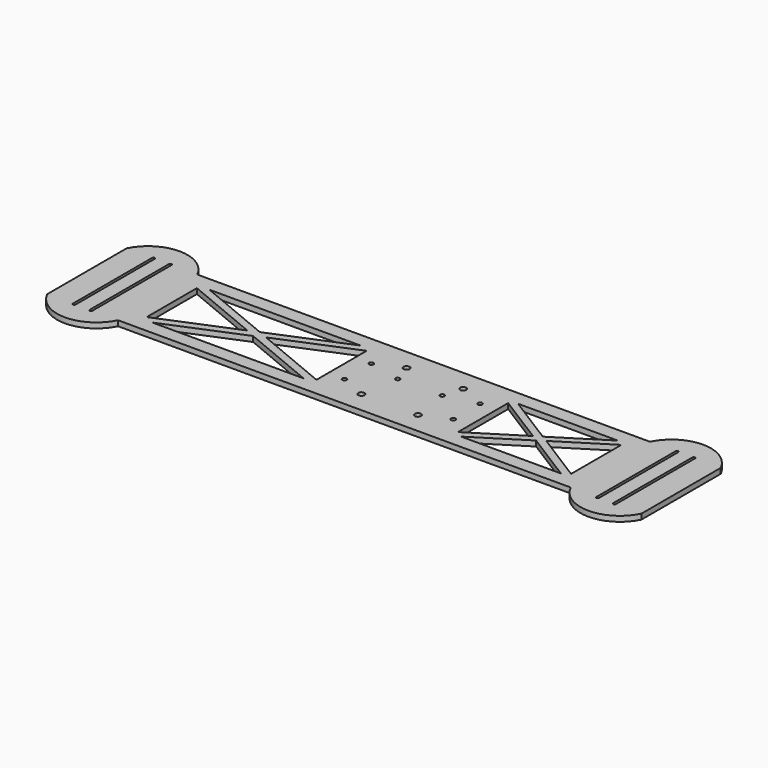
from build123d import *

# Parameters (mm, degrees)
F1_DEPTH = 4.7625
F3_D     = 11.1125
F4_D     = 7.9375


# Not quite as in the source:
# - a length typed as a fraction of an inch, garbled in the dataset ("3 / 203.2 mm" for 3/8 in), is restored


with BuildPart() as f1:
    # F0 (on Top) → F1 (new body, symmetric)
    with BuildSketch(Plane.XY):
        with BuildLine():
            ThreePointArc((533.4, 88.9), (469.9, 128.5875), (406.4, 88.9))
            Line((406.4, 88.9), (-406.4, 88.9))
            ThreePointArc((-406.4, 88.9), (-469.9, 128.5875), (-533.4, 88.9))
            Line((-533.4, 88.9), (-533.4, -88.9))
            ThreePointArc((-533.4, -88.9), (-469.9, -128.5875), (-406.4, -88.9))
            Line((-406.4, -88.9), (406.4, -88.9))
            ThreePointArc((406.4, -88.9), (469.9, -128.5875), (533.4, -88.9))
            Line((533.4, -88.9), (533.4, 88.9))
        make_face()
        Polygon((-364.33125, -64.29375), (-228.6, -7.9375), (-92.86875, -64.29375), align=None, mode=Mode.SUBTRACT)
        Polygon((189.70625, -64.29375), (279.4, -7.9375), (369.09375, -64.29375), align=None, mode=Mode.SUBTRACT)
        with BuildLine():
            ThreePointArc((-487.3625, 88.9), (-484.98125, 91.28125), (-482.6, 88.9))
            Line((-482.6, 88.9), (-482.6, -88.9))
            ThreePointArc((-482.6, -88.9), (-484.98125, -91.28125), (-487.3625, -88.9))
            Line((-487.3625, -88.9), (-487.3625, 88.9))
        make_face(mode=Mode.SUBTRACT)
        with BuildLine():
            ThreePointArc((-457.2, 88.9), (-454.81875, 91.28125), (-452.4375, 88.9))
            Line((-452.4375, 88.9), (-452.4375, -88.9))
            ThreePointArc((-452.4375, -88.9), (-454.81875, -91.28125), (-457.2, -88.9))
            Line((-457.2, -88.9), (-457.2, 88.9))
        make_face(mode=Mode.SUBTRACT)
        Polygon((-381, -56.35625), (-381, 56.35625), (-245.26875, 0), align=None, mode=Mode.SUBTRACT)
        Polygon((-76.2, -56.35625), (-211.93125, 0), (-76.2, 56.35625), align=None, mode=Mode.SUBTRACT)
        Polygon((-92.86875, 63.5), (-228.6, 7.14375), (-364.33125, 63.5), align=None, mode=Mode.SUBTRACT)
        Polygon((177.8, 56.35625), (267.49375, 0), (177.8, -56.35625), align=None, mode=Mode.SUBTRACT)
        Polygon((291.30625, 0), (381, 56.35625), (381, -56.35625), align=None, mode=Mode.SUBTRACT)
        with BuildLine():
            Line((452.4375, -88.9), (452.4375, 88.9))
            ThreePointArc((452.4375, 88.9), (454.81875, 91.28125), (457.2, 88.9))
            Line((457.2, 88.9), (457.2, -88.9))
            ThreePointArc((457.2, -88.9), (454.81875, -91.28125), (452.4375, -88.9))
        make_face(mode=Mode.SUBTRACT)
        with BuildLine():
            ThreePointArc((487.3625, -88.9), (484.98125, -91.28125), (482.6, -88.9))
            Line((482.6, -88.9), (482.6, 88.9))
            ThreePointArc((482.6, 88.9), (484.98125, 91.28125), (487.3625, 88.9))
            Line((487.3625, 88.9), (487.3625, -88.9))
        make_face(mode=Mode.SUBTRACT)
        Polygon((369.09375, 63.5), (279.4, 7.14375), (189.70625, 63.5), align=None, mode=Mode.SUBTRACT)
    extrude(amount=F1_DEPTH, both=True)

    # F3 (through all)
    with Locations(Plane.XY.offset(4.7625)):
        with Locations((0, 50.8), (101.6, 50.8), (101.6, -50.8), (0, -50.8)):
            Hole(F3_D / 2)

    # F4 (through all)
    with Locations(Plane.XY.offset(4.7625)):
        with Locations((-46.83125, 30.1625), (-46.83125, -30.1625), (11.1125, 16.69415), (91.28125, 16.69415), (148.43125, 30.1625), (148.43125, -30.1625)):
            Hole(F4_D / 2)


solid = f1.part
